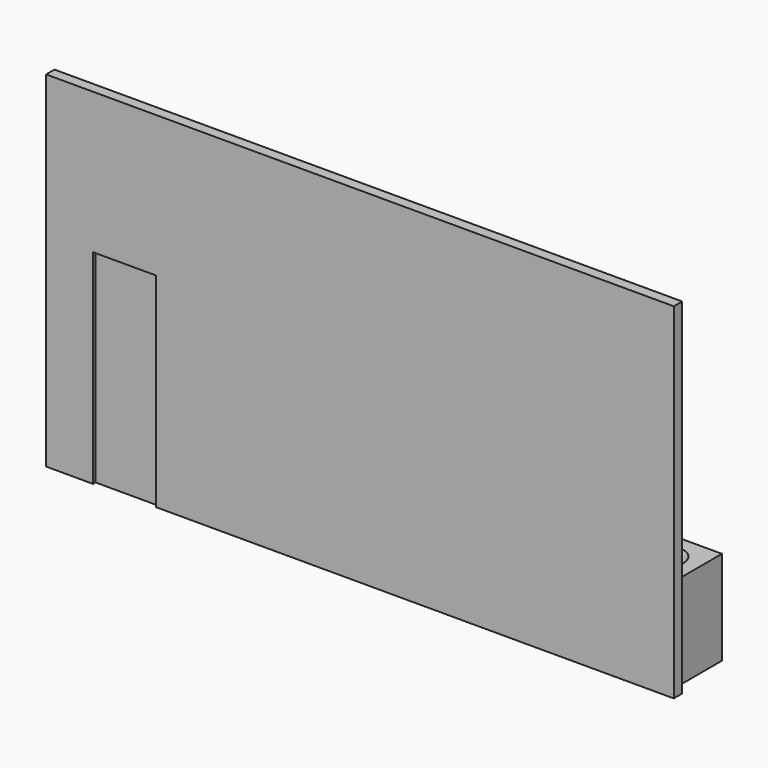
from build123d import *

# Parameters (mm, degrees)
F0_W         = 6096
F0_H         = 3352.8
F1_DEPTH     = 101.6
F2_W         = 609.6
F2_H         = 1981.2
F3_DEPTH     = 30.48
F4_W         = 609.6
F4_H         = 1981.2
F5_DEPTH     = 30.48
F7_DEPTH     = 685.8
F9_DEPTH     = 609.6
F6_W         = 609.6
F6_H         = 914.4
F10_DEPTH    = 609.6
F11_R        = 176.6748318238
F12_DEPTH    = 76.2
F14_W        = 431.8
F14_H        = 609.6
F15_DEPTH    = 25.4
F16_W        = 431.8
F16_H        = 330.2
F17_DEPTH    = 203.2
F19_DEPTH    = 25.4
F6_W_2       = 584.2
F6_H_2       = 762
F20_DEPTH    = 25.4
F21_T1_DEPTH = 1009.5685763581
F21_T3_DEPTH = 707.9842881791


# Not quite as in the source:
# - a fillet or chamfer that OpenCascade refuses, or shapes differently, is made with other operations: its cross-section is extruded or revolved along the edge and cut away or added


with BuildPart() as f1:
    # F0 (on Front) → F1 (new body)
    with BuildSketch(Plane.XZ):
        with Locations((-3048, 1676.4)):
            Rectangle(F0_W, F0_H)
    extrude(amount=F1_DEPTH)

    # F2 (on face) → F3 (cut)
    with BuildSketch(Plane.XZ.offset(101.6)):
        with Locations((-5334, 990.6)):
            Rectangle(F2_W, F2_H)
    extrude(amount=-F3_DEPTH, mode=Mode.SUBTRACT)

    # F4 (on face) → F5 (cut)
    with BuildSketch(Plane(origin=(0, 0, 0), x_dir=(-1, 0, 0), z_dir=(0, 1, 0))):
        with Locations((5334, 990.6)):
            Rectangle(F4_W, F4_H)
    extrude(amount=-F5_DEPTH, mode=Mode.SUBTRACT)

    # F6 (on face) → F7 (join)
    with BuildSketch(Plane(origin=(0, 0, 0), x_dir=(-1, 0, 0), z_dir=(0, 1, 0))):
        Polygon((711.2, 914.4), (711.2, 0), (1295.4, 0), (1295.4, 1828.8), (711.2, 1828.8), align=None)
    extrude(amount=F7_DEPTH)

    # F8 (on face) → F9 (cut)
    with BuildSketch(Plane.YZ.offset(-711.2)):
        Polygon((203.2, 762), (685.8, 762), (685.8, 1066.8), align=None)
    extrude(amount=-F9_DEPTH, mode=Mode.SUBTRACT)

    # F6 (on face) → F10 (join)
    with BuildSketch(Plane(origin=(0, 0, 0), x_dir=(-1, 0, 0), z_dir=(0, 1, 0))):
        with Locations((406.4, 457.2)):
            Rectangle(F6_W, F6_H)
    extrude(amount=F10_DEPTH)

    # F11 (on face) → F12 (cut)
    with BuildSketch(Plane.XY.offset(914.4)):
        with Locations((-408.9462161064, 304.8)):
            Circle(F11_R)
    extrude(amount=-F12_DEPTH, mode=Mode.SUBTRACT)

    # F13: fillet of radius 127 on 1 edges, made by hand

    # F13_s1 → F13_t2 (revolve)
    with BuildSketch(Plane.XZ.offset(-304.8)):
        with BuildLine():
            ThreePointArc((-232.2713842826, 914.4), (-279.1080421313, 858.9441766302), (-348.6688069344, 838.2))
            Line((-348.6688069344, 838.2), (-232.2713842826, 838.2))
            Line((-232.2713842826, 838.2), (-232.2713842826, 914.4))
        make_face()
    revolve(axis=Axis((-408.9462161064, 304.8, 838.2), (0, 0, 1)))

    # F14 (on face) → F15 (join)
    with BuildSketch(Plane(origin=(0, 685.8, 0), x_dir=(-1, 0, 0), z_dir=(0, 1, 0))):
        with Locations((1003.3, 1447.8)):
            Rectangle(F14_W, F14_H)
    extrude(amount=F15_DEPTH)

    # F16 (on face) → F17 (cut)
    with BuildSketch(Plane.XY.offset(762)):
        with Locations((-1003.3, 444.5)):
            Rectangle(F16_W, F16_H)
    extrude(amount=-F17_DEPTH, mode=Mode.SUBTRACT)

    # F18 (on face) → F19 (join)
    with BuildSketch(Plane(origin=(0, 609.6, 0), x_dir=(-1, 0, 0), z_dir=(0, 1, 0))):
        Polygon((152.4, 50.8), (660.4, 50.8), (660.4, 762), (660.4, 863.6), (152.4, 863.6), align=None)
    extrude(amount=F19_DEPTH)

    # F6 (on face) → F20 (join)
    with BuildSketch(Plane(origin=(0, 0, 0), x_dir=(-1, 0, 0), z_dir=(0, 1, 0))):
        with Locations((393.7, 1447.8)):
            Rectangle(F6_W_2, F6_H_2)
    extrude(amount=F20_DEPTH)

    # F21: fillet of radius 60.96 on 4 edges, made by hand

    # F21_s2 → F21_t1 (cut)
    with BuildSketch(Plane.XY.offset(943.0157118209)):
        with BuildLine():
            ThreePointArc((-101.6, 0), (-123.2894093504, 18.6795575203), (-151.1137152716, 25.4))
            Line((-151.1137152716, 25.4), (-101.6, 25.4))
            Line((-101.6, 25.4), (-101.6, 0))
        make_face()
        with BuildLine():
            ThreePointArc((-685.8, 0), (-664.1105906496, 18.6795575203), (-636.2862847284, 25.4))
            Line((-636.2862847284, 25.4), (-685.8, 25.4))
            Line((-685.8, 25.4), (-685.8, 0))
        make_face()
    extrude(amount=F21_T1_DEPTH, mode=Mode.SUBTRACT)

    # F21_s4 → F21_t3 (cut)
    with BuildSketch(Plane.YZ.offset(-685.8)):
        with BuildLine():
            ThreePointArc((0, 1066.8), (18.6795575203, 1088.4894093504), (25.4, 1116.3137152716))
            Line((25.4, 1116.3137152716), (25.4, 1066.8))
            Line((25.4, 1066.8), (0, 1066.8))
        make_face()
        with BuildLine():
            ThreePointArc((0, 1828.8), (18.6795575203, 1807.1105906496), (25.4, 1779.2862847284))
            Line((25.4, 1779.2862847284), (25.4, 1828.8))
            Line((25.4, 1828.8), (0, 1828.8))
        make_face()
    extrude(amount=F21_T3_DEPTH, mode=Mode.SUBTRACT)


solid = f1.part
